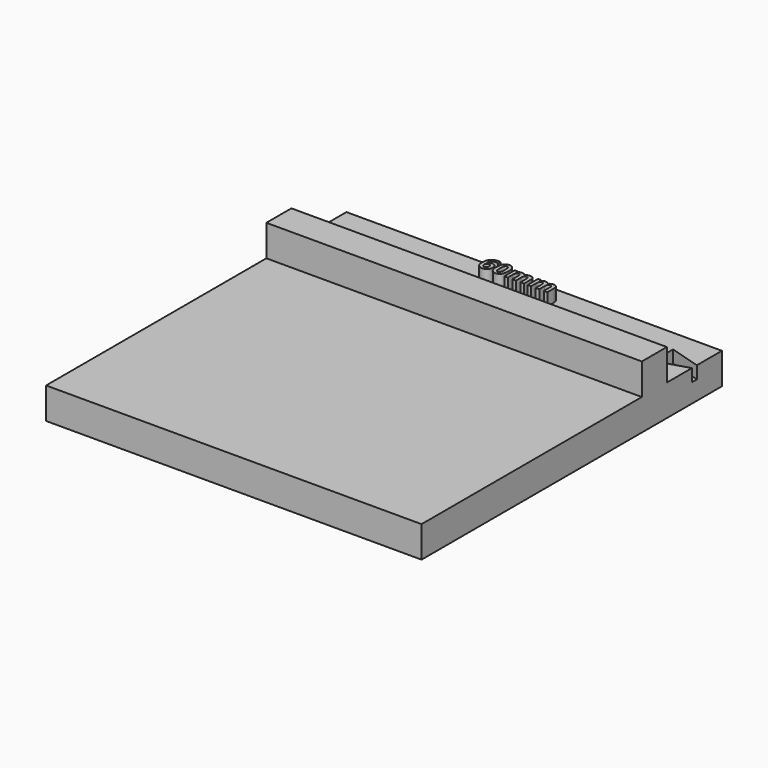
from build123d import *

# Parameters (mm, degrees)
F0_W         = 60
F0_H         = 60
F1_DEPTH     = 5
F3_DEPTH     = 2
F4_DEPTH     = 2
F5_TEXT_SIZE = 3.8052727986
F6_DEPTH     = 2
F8_DEPTH     = 5


# Not quite as in the source:
# - Text() gives the source's letters only with a copy of the font that has no kerning and outlines rounded to 1/6400 em; it was checked with that copy


with BuildPart() as f1:
    # F0 (on Top) → F1 (new body)
    with BuildSketch(Plane.XY):
        Rectangle(F0_W, F0_H)
    extrude(amount=F1_DEPTH)

    # F2 (on face) → F3 (cut)
    with BuildSketch(Plane.XY.offset(5)):
        Polygon((25, 25), (0, 25), (-25, 25), (-25, 26.5), (-30, 25), (-30, 24), (-25, 22.5), (-25, 24), (0, 24), (25, 24), (25, 22.5), (30, 24), (30, 25), (25, 26.5), align=None)
    extrude(amount=-F3_DEPTH, mode=Mode.SUBTRACT)

    # F2 (on face) → F4 (cut)
    with BuildSketch(Plane.XY.offset(5)):
        Polygon((25, 25), (0, 25), (-25, 25), (-25, 26.5), (-30, 25), (-30, 24), (-25, 22.5), (-25, 24), (0, 24), (25, 24), (25, 22.5), (30, 24), (30, 25), (25, 26.5), align=None)
    extrude(amount=-F4_DEPTH, mode=Mode.SUBTRACT)

    # F5 (on face) → F6 (join)
    with BuildSketch(Plane.XY.offset(5)):
        with Locations((-6.027654279, 25.757972151)):
            Text('60mm', F5_TEXT_SIZE, font='Open Sans', font_style=FontStyle.BOLD, text_align=(TextAlign.LEFT, TextAlign.BOTTOM))
    extrude(amount=F6_DEPTH)

    # F7 (on face) → F8 (join)
    with BuildSketch(Plane.XY.offset(5)):
        Polygon((-30, 14), (0, 14), (30, 14), (30, 19), (-30, 19), align=None)
    extrude(amount=F8_DEPTH)


solid = f1.part
